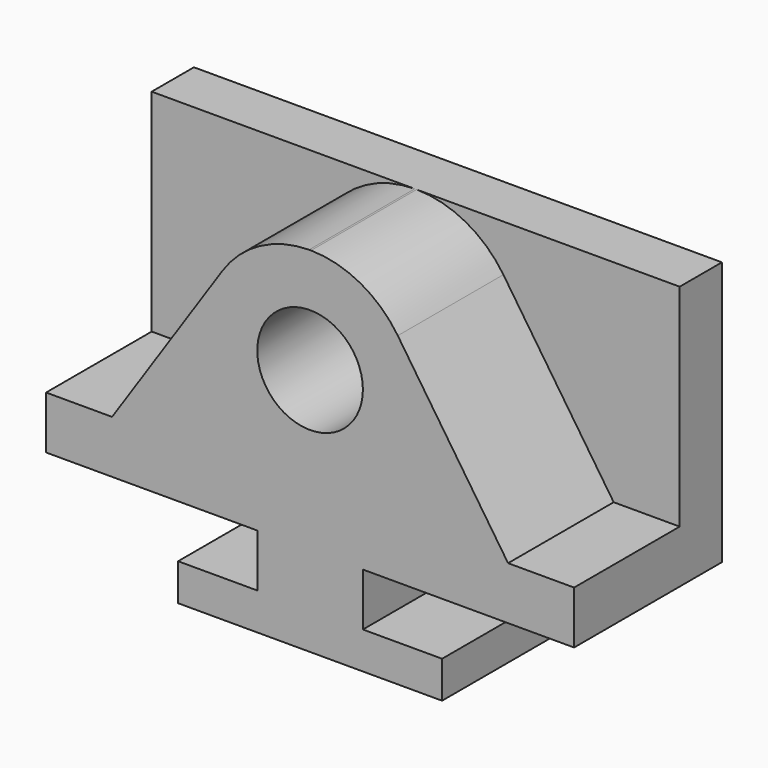
from build123d import *

# Parameters (mm, degrees)
F0_R     = 12.7
F1_DEPTH = 44.45
F2_DEPTH = 12.7


with BuildPart() as f1:
    # F0 (on Front) → F1 (new body)
    with BuildSketch(Plane.XZ):
        with BuildLine():
            Line((-31.75, 0), (0, 0))
            Line((0, 0), (31.75, 0))
            Line((31.75, 0), (31.75, 8.89))
            Line((31.75, 8.89), (12.7, 8.89))
            Line((12.7, 8.89), (12.7, 21.59))
            Line((12.7, 21.59), (63.5, 21.59))
            Line((63.5, 21.59), (63.5, 34.29))
            Line((63.5, 34.29), (47.625, 34.29))
            Line((47.625, 34.29), (21.0935941582, 73.8409400841))
            ThreePointArc((21.0935941582, 73.8409400841), (12.0532981257, 82.0489700372), (0.2274431955, 85.09))
            Line((0.2274431955, 85.09), (-0.2274431955, 85.09))
            ThreePointArc((-0.2274431955, 85.09), (-12.0532981257, 82.0489700372), (-21.0935941582, 73.8409400841))
            Line((-21.0935941582, 73.8409400841), (-47.625, 34.29))
            Line((-47.625, 34.29), (-63.5, 34.29))
            Line((-63.5, 34.29), (-63.5, 21.59))
            Line((-63.5, 21.59), (-12.7, 21.59))
            Line((-12.7, 21.59), (-12.7, 8.89))
            Line((-12.7, 8.89), (-31.75, 8.89))
            Line((-31.75, 8.89), (-31.75, 0))
        make_face()
        with Locations((0, 59.6910183355)):
            Circle(F0_R, mode=Mode.SUBTRACT)
    extrude(amount=F1_DEPTH)

    # F0 (on Front) → F2 (join)
    with BuildSketch(Plane.XZ):
        with BuildLine():
            Line((-31.75, 0), (0, 0))
            Line((0, 0), (31.75, 0))
            Line((31.75, 0), (31.75, 8.89))
            Line((31.75, 8.89), (12.7, 8.89))
            Line((12.7, 8.89), (12.7, 21.59))
            Line((12.7, 21.59), (63.5, 21.59))
            Line((63.5, 21.59), (63.5, 34.29))
            Line((63.5, 34.29), (47.625, 34.29))
            Line((47.625, 34.29), (21.0935941582, 73.8409400841))
            ThreePointArc((21.0935941582, 73.8409400841), (12.0532981257, 82.0489700372), (0.2274431955, 85.09))
            Line((0.2274431955, 85.09), (-0.2274431955, 85.09))
            ThreePointArc((-0.2274431955, 85.09), (-12.0532981257, 82.0489700372), (-21.0935941582, 73.8409400841))
            Line((-21.0935941582, 73.8409400841), (-47.625, 34.29))
            Line((-47.625, 34.29), (-63.5, 34.29))
            Line((-63.5, 34.29), (-63.5, 21.59))
            Line((-63.5, 21.59), (-12.7, 21.59))
            Line((-12.7, 21.59), (-12.7, 8.89))
            Line((-12.7, 8.89), (-31.75, 8.89))
            Line((-31.75, 8.89), (-31.75, 0))
        make_face()
        with Locations((0, 59.6910183355)):
            Circle(F0_R, mode=Mode.SUBTRACT)
        with BuildLine():
            Line((47.625, 34.29), (63.5, 34.29))
            Line((63.5, 34.29), (63.5, 85.09))
            Line((63.5, 85.09), (0.2274431955, 85.09))
            ThreePointArc((0.2274431955, 85.09), (12.0532981257, 82.0489700372), (21.0935941582, 73.8409400841))
            Line((21.0935941582, 73.8409400841), (47.625, 34.29))
        make_face()
        with BuildLine():
            Line((-63.5, 85.09), (-63.5, 34.29))
            Line((-63.5, 34.29), (-47.625, 34.29))
            Line((-47.625, 34.29), (-21.0935941582, 73.8409400841))
            ThreePointArc((-21.0935941582, 73.8409400841), (-12.0532981257, 82.0489700372), (-0.2274431955, 85.09))
            Line((-0.2274431955, 85.09), (-63.5, 85.09))
        make_face()
    extrude(amount=F2_DEPTH)


solid = f1.part
